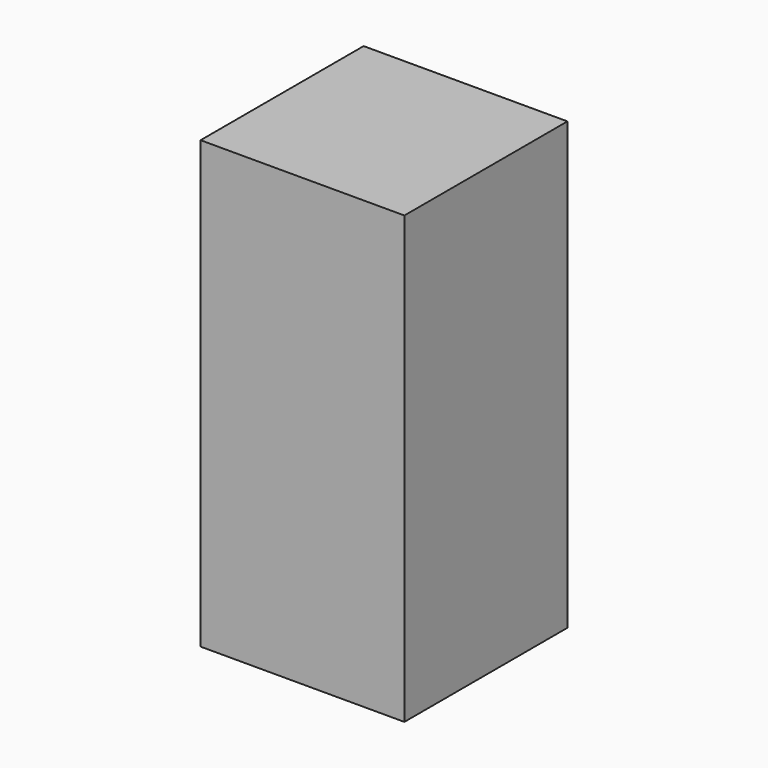
from build123d import *

# Parameters (mm, degrees)
F0_W     = 16
F0_H     = 10
F1_DEPTH = 16
F2_W     = 14
F2_H     = 14
F2_R     = 3.25
F2_R_2   = 2.75
F3_DEPTH = 8.5
F5_DEPTH = 25
F4_R     = 2.5
F6_DEPTH = 2


# Not quite as in the source:
# - a feature names something its author has since deleted; it is built from what else it names


with BuildPart() as f1:
    # F0 (on Right) → F1 (new body)
    with BuildSketch(Plane.YZ):
        with Locations((0.4982002154, -0.3821941838)):
            Rectangle(F0_W, F0_H)
    extrude(amount=F1_DEPTH)

    # F2 (on face) → F3 (cut)
    with BuildSketch(Plane(origin=(0, 0, -5.3821941838), x_dir=(1, 0, 0), z_dir=(0, 0, -1))):
        with Locations((8, -0.4982002154)):
            Rectangle(F2_W, F2_H)
        with Locations((8, 0)):
            Circle(F2_R, mode=Mode.SUBTRACT)
        with Locations((8, 0)):
            Circle(F2_R_2)
    extrude(amount=-F3_DEPTH, mode=Mode.SUBTRACT)

    # F5 (add): a face of the model
    f5_faces = [f1.faces().sort_by_distance(p)[0] for p in [
        (8, 0.4982002154, 4.6178058162),
    ]]
    extrude(f5_faces, amount=F5_DEPTH)

    # F4 (on Top) → F6, piece 3 (join)
    with BuildSketch(Plane.XY):
        with Locations((4, -4.4982002154)):
            Circle(F4_R)
        with Locations((12, -4.4982002154)):
            Circle(F4_R)
    extrude(amount=-F6_DEPTH)


with BuildPart() as f6:
    # F4 (on Top) → F6 (new body)
    with BuildSketch(Plane.XY):
        with Locations((4, 4.4982002154)):
            Circle(F4_R)
    extrude(amount=-F6_DEPTH)


with BuildPart() as f6b:
    # F4 (on Top) → F6, piece 2 (new body)
    with BuildSketch(Plane.XY):
        with Locations((12, 4.4982002154)):
            Circle(F4_R)
    extrude(amount=-F6_DEPTH)


solid = Compound([f1.part, f6.part, f6b.part])
